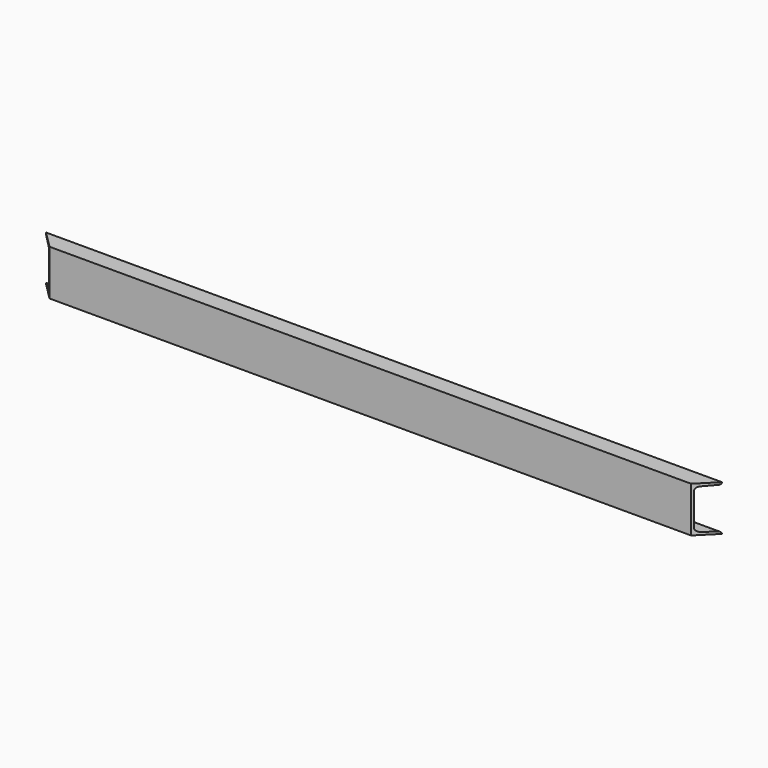
from build123d import *

# Parameters (mm, degrees)
F1_DEPTH = 3000
F3_DEPTH = 203.001


# Not quite as in the source:
# - a pattern or mirror of a feature is missing from the dataset's text; its kind, count and spacing are read off the source's solid


with BuildPart() as f1:
    # F0 (on Right) → F1 (new body)
    with BuildSketch(Plane.YZ):
        with BuildLine():
            Line((0, 203), (0, 0.7243087391))
            Line((0, 0.7243087391), (76, 0.7243087391))
            Line((76, 0.7243087391), (76, 2.0526619257))
            ThreePointArc((76, 2.0526619257), (73.6656821536, 7.9036758191), (67.9448556281, 10.5410129711))
            Line((67.9448556281, 10.5410129711), (23.2102887439, 12.8854522787))
            ThreePointArc((23.2102887439, 12.8854522787), (11.7686356928, 18.1601265828), (7.1, 29.8621543695))
            Line((7.1, 29.8621543695), (7.1, 173.8621543695))
            ThreePointArc((7.1, 173.8621543695), (11.7686356928, 185.5641821563), (23.2102887439, 190.8388564604))
            Line((23.2102887439, 190.8388564604), (67.9448556281, 193.183295768))
            ThreePointArc((67.9448556281, 193.183295768), (73.6656821536, 195.82063292), (76, 201.6716468134))
            Line((76, 201.6716468134), (76, 203))
            Line((76, 203), (0, 203))
        make_face()
    extrude(amount=F1_DEPTH)

    # F2 (on Top) → F3 (cut, through all)
    with BuildSketch(Plane.XY):
        Polygon((0, 76), (0, 0), (76, 0), align=None)
    f3 = extrude(amount=F3_DEPTH, mode=Mode.SUBTRACT)

    # F3_copies: F3 across plane
    add(f3.mirror(Plane(origin=(1500, 0, 0), x_dir=(0, 0, 1), z_dir=(1, 0, 0))), mode=Mode.SUBTRACT)


solid = f1.part
